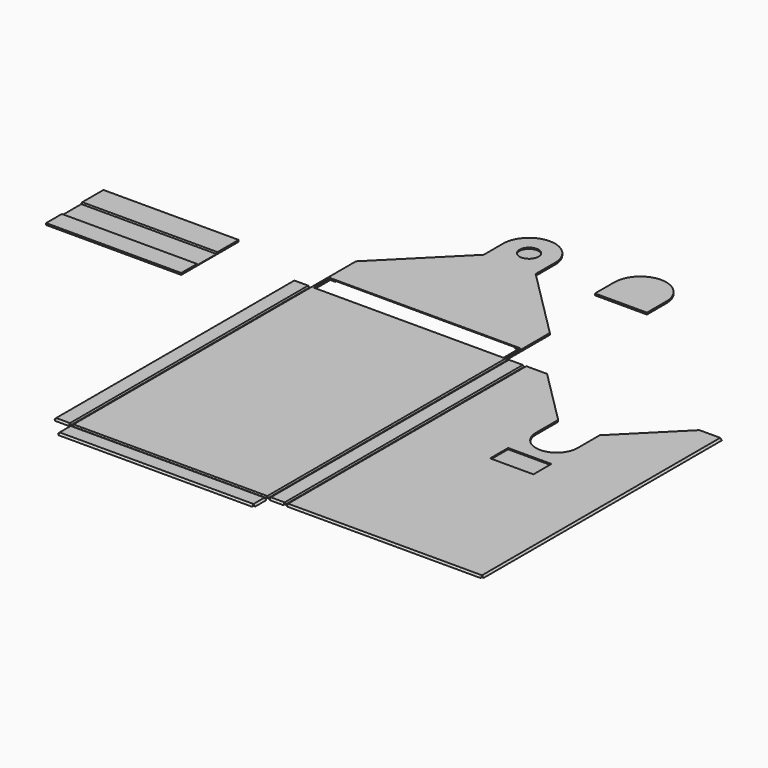
from build123d import *

# Parameters (mm, degrees)
F0_W      = 56
F0_H      = 8
F0_H_2    = 86
F0_W_2    = 0.5
F0_H_3    = 0.5
F0_H_4    = 43
F0_W_3    = 4
F0_H_5    = 4
F1_DEPTH  = 0.5
F2_SIZE2  = 0.49999
F2_SIZE   = 0.49999
F4_DEPTH  = 86
F6_DEPTH  = 25
F7_R      = 2.75
F8_DEPTH  = 0.35
F9_W      = 12.5
F9_H      = 6.5
F10_DEPTH = 0.35
F11_W     = 39.043193683
F11_H     = 5.6905061938
F11_H_2   = 7.6418016106
F11_H_3   = 7.3748123832
F12_DEPTH = 0.15
F13_DEPTH = 0.5
F14_SIZE  = 0.34999
F15_W     = 54.8
F15_H     = 6
F16_DEPTH = 25
F17_R     = 5.99999
F18_SIZE  = 16
F20_DEPTH = 56
F22_DEPTH = 0.5
F25_DEPTH = 0.25


# Not quite as in the source:
# - a fillet or chamfer is up to 0.001 mm smaller than in the source, because OpenCascade refuses the exact size


with BuildPart() as f1:
    # F0 (on Top) → F1 (new body)
    with BuildSketch(Plane.XY):
        with Locations((28, 4)):
            Rectangle(F0_W, F0_H)
        with Locations((28, -43)):
            Rectangle(F0_W, F0_H_2)
        with Locations((-0.25, -43)):
            Rectangle(F0_W_2, F0_H_2)
        with Locations((56.25, -43)):
            Rectangle(F0_W_2, F0_H_2)
        with Locations((28, -86.25)):
            Rectangle(F0_W, F0_H_3)
        with Locations((-0.75, -43)):
            Rectangle(F0_W_2, F0_H_2)
        with Locations((28, 29.5)):
            Rectangle(F0_W, F0_H_4)
        with Locations((56.75, -43)):
            Rectangle(F0_W_2, F0_H_2)
        with Locations((28, -86.75)):
            Rectangle(F0_W, F0_H_3)
        with Locations((-3, -43)):
            Rectangle(F0_W_3, F0_H_2)
        with Locations((59, -43)):
            Rectangle(F0_W_3, F0_H_2)
        with Locations((-3, -86.25)):
            Rectangle(F0_W_3, F0_H_3)
        with Locations((28, -89)):
            Rectangle(F0_W, F0_H_5)
        with Locations((-0.25, -89)):
            Rectangle(F0_W_2, F0_H_5)
        with Locations((-5.25, -43)):
            Rectangle(F0_W_2, F0_H_2)
        with Locations((59, -86.25)):
            Rectangle(F0_W_3, F0_H_3)
        with Locations((56.25, -89)):
            Rectangle(F0_W_2, F0_H_5)
        with Locations((61.25, -43)):
            Rectangle(F0_W_2, F0_H_2)
        with Locations((28, -91.25)):
            Rectangle(F0_W, F0_H_3)
        with Locations((61.75, -43)):
            Rectangle(F0_W_2, F0_H_2)
        Polygon((84, 0), (62, 0), (62, -86), (118, -86), (118, 0), (96, 0), (96, -30), (84, -30), align=None)
        with Locations((90, -86.25)):
            Rectangle(F0_W, F0_H_3)
        with Locations((118.25, -43)):
            Rectangle(F0_W_2, F0_H_2)
    extrude(amount=F1_DEPTH)

    # F2 (size 0.5 and 0.5 in the source; OpenCascade refuses exactly that, so slightly less here)
    f2_edges = [f1.edges().sort_by_distance(p)[0] for p in [
        (-5.5, -43, 0.5),
        (-3, -86.5, 0.5),
        (-0.5, -89, 0.5),
        (28, -91.5, 0.5),
        (56.5, -89, 0.5),
        (59, -86.5, 0.5),
        (90, -86.5, 0.5),
        (118.5, -43, 0.5),
    ]]
    chamfer(f2_edges, length=F2_SIZE, length2=F2_SIZE2)

    # F3 (on face) → F4 (cut, through all)
    with BuildSketch(Plane.XZ.offset(86)):
        Polygon((0, 0.5), (-1, 0.5), (-0.65, 0.15), (-0.35, 0.15), align=None)
        Polygon((57, 0.5), (56, 0.5), (56.35, 0.15), (56.65, 0.15), align=None)
        Polygon((62, 0.5), (61, 0.5), (61.35, 0.15), (61.65, 0.15), align=None)
    extrude(amount=-F4_DEPTH, mode=Mode.SUBTRACT)

    # F5 (on face) → F6 (cut)
    with BuildSketch(Plane.XY.offset(0.5)):
        with BuildLine():
            Line((34, 51), (28, 51))
            ThreePointArc((28, 51), (33.3033008589, 48.8033008589), (35.5, 43.5))
            Line((35.5, 43.5), (35.5, 36.5))
            Line((35.5, 36.5), (56, 16))
            Line((56, 16), (56, 51))
            Line((56, 51), (34, 51))
        make_face()
        with BuildLine():
            Line((28, 51), (22, 51))
            Line((22, 51), (0, 51))
            Line((0, 51), (0, 16))
            Line((0, 16), (20.5, 36.5))
            Line((20.5, 36.5), (20.5, 43.5))
            ThreePointArc((20.5, 43.5), (22.6966991411, 48.8033008589), (28, 51))
        make_face()
    extrude(amount=-F6_DEPTH, mode=Mode.SUBTRACT)

    # F7 (on face) → F8 (cut)
    with BuildSketch(Plane.XY.offset(0.5)):
        with Locations((28, 43.5)):
            Circle(F7_R)
    extrude(amount=-F8_DEPTH, mode=Mode.SUBTRACT)

    # F9 (on face) → F10 (cut)
    with BuildSketch(Plane.XY.offset(0.5)):
        with Locations((90, -37)):
            Rectangle(F9_W, F9_H)
    extrude(amount=-F10_DEPTH, mode=Mode.SUBTRACT)

    # F15 (on face) → F16 (cut)
    with BuildSketch(Plane.XY.offset(0.5)):
        with Locations((28, 3)):
            Rectangle(F15_W, F15_H)
    extrude(amount=-F16_DEPTH, mode=Mode.SUBTRACT)

    # F17 (radius 6 in the source; OpenCascade refuses exactly that, so slightly less here)
    f17_edges = [f1.edges().sort_by_distance(p)[0] for p in [
        (84, -30, 0.25),
        (96, -30, 0.25),
    ]]
    fillet(f17_edges, radius=F17_R)

    # F18
    f18_edges = [f1.edges().sort_by_distance(p)[0] for p in [
        (84, 0, 0.25),
        (96, 0, 0.25),
    ]]
    chamfer(f18_edges, length=F18_SIZE)

    # F19 (on face) → F20 (cut, through all)
    with BuildSketch(Plane.YZ.offset(56)):
        Polygon((-86, 0.5), (-87, 0.5), (-86.65, 0.15), (-86.35, 0.15), align=None)
    extrude(amount=-F20_DEPTH, mode=Mode.SUBTRACT)

    # F24 (on face) → F25 (cut)
    with BuildSketch(Plane(origin=(0, 0, 0), x_dir=(1, 0, 0), z_dir=(0, 0, -1))):
        with BuildLine():
            Line((54, -15.1715728753), (54, 38.8284271247))
            ThreePointArc((54, 38.8284271247), (51.6568542495, 44.4852813742), (46, 46.8284271247))
            Line((46, 46.8284271247), (10, 46.8284271247))
            ThreePointArc((10, 46.8284271247), (4.3431457505, 44.4852813742), (2, 38.8284271247))
            Line((2, 38.8284271247), (2, -15.1715728753))
            Line((2, -15.1715728753), (21.3284271247, -34.5))
            Line((21.3284271247, -34.5), (34.6715728753, -34.5))
            Line((34.6715728753, -34.5), (54, -15.1715728753))
        make_face()
    extrude(amount=-F25_DEPTH, mode=Mode.SUBTRACT)


with BuildPart() as f12:
    # F11 (on Top) → F12 (new body)
    with BuildSketch(Plane.XY):
        with Locations((-46.7307167128, -10.2200654801)):
            Rectangle(F11_W, F11_H)
        with Locations((-46.7307167128, 3.8209008053)):
            Rectangle(F11_W, F11_H_2)
        with Locations((-46.7307167128, -3.6874061916)):
            Rectangle(F11_W, F11_H_3)
    extrude(amount=F12_DEPTH)

    # F11 (on Top) → F13 (join)
    with BuildSketch(Plane.XY):
        with Locations((-46.7307167128, -10.2200654801)):
            Rectangle(F11_W, F11_H)
        with Locations((-46.7307167128, 3.8209008053)):
            Rectangle(F11_W, F11_H_2)
    extrude(amount=F13_DEPTH)

    # F14 (size 0.35 in the source; OpenCascade refuses exactly that, so slightly less here)
    f14_edges = [f12.edges().sort_by_distance(p)[0] for p in [
        (-46.730717, -7.374812, 0.15),
        (-46.730717, 0, 0.15),
    ]]
    chamfer(f14_edges, length=F14_SIZE)


with BuildPart() as f22:
    # F21 (on Top) → F22 (new body)
    with BuildSketch(Plane.XY):
        with BuildLine():
            Line((51.8908984959, 44.4321229756), (51.8908984959, 37.4321229756))
            Line((51.8908984959, 37.4321229756), (66.8908984959, 37.4321229756))
            Line((66.8908984959, 37.4321229756), (66.8908984959, 44.4321229756))
            ThreePointArc((66.8908984959, 44.4321229756), (59.3908984959, 51.9321229756), (51.8908984959, 44.4321229756))
        make_face()
    extrude(amount=F22_DEPTH)


solid = Compound([f1.part, f12.part, f22.part])
